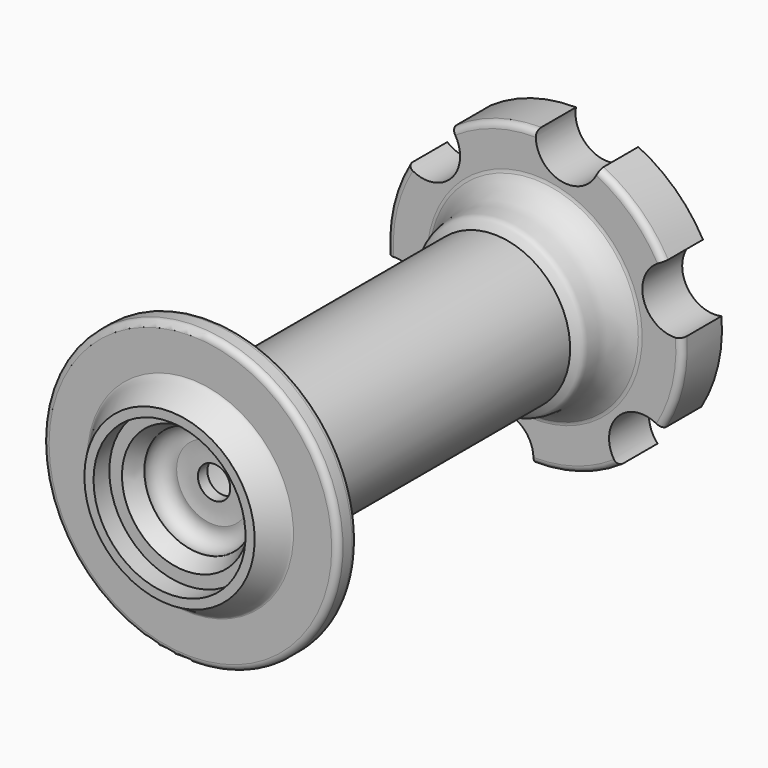
from build123d import *

# Parameters (mm, degrees)
F2_R          = 1
F4_R          = 5.0872245557
F5_DEPTH      = 25
F5_DEPTH_BACK = 25


# Not quite as in the source:
# - a feature names something its author has since deleted; it is built from what else it names


with BuildPart() as f1:
    # F0 (on Top) → F1 (revolve)
    with BuildSketch(Plane.XY):
        with BuildLine():
            Line((-12.045, 24.19), (-12.045, 0))
            Line((-12.045, 0), (-12.045, -24.19))
            add(Edge.make_bspline(
                [(-12.045, -24.19), (-12.5958616321, -24.4968671697), (-13.7960381357, -25.0826911965), (-13.4774444038, -27.9229008757), (-15.2810031254, -31.3268076458), (-16.4584506699, -32.0230348179), (-16.8, -32.2)],
                knots=[0, 0, 0, 0, 0.2130240833, 0.4757651617, 0.7943682617, 1, 1, 1, 1], degree=3))
            Line((-16.8, -32.2), (-23.4, -32.2))
            Line((-23.4, -32.2), (-23.4, -36))
            Line((-23.4, -36), (-16.34, -36))
            add(Edge.make_bspline(
                [(-16.34, -36), (-16.0707529319, -35.9620323671), (-14.9726425226, -37.6439271493), (-14.3452255143, -38.6538248832), (-13.7752974798, -39.6449017449), (-13.5, -40.14)],
                knots=[0, 0, 0, 0, 0.3581062946, 0.6698519127, 1, 1, 1, 1], degree=3))
            Line((-13.5, -40.14), (-12.045, -40.14))
            Line((-12.045, -40.14), (-12.045, -37.01))
            Line((-12.045, -37.01), (-10.045, -37.01))
            add(Edge.make_bspline(
                [(-10.045, -37.01), (-9.4132699561, -35.9848800804), (-9.0350072413, -35.0615949654), (-8.684367441, -34.2704410489)],
                knots=[0, 0, 0, 0, 2.6156118111, 2.6156118111, 2.6156118111, 2.6156118111], degree=3))
            ThreePointArc((-8.684367441, -34.2704410489), (-8.0143701637, -32.0764184583), (-5.8012267005, -31.4725745291))
            add(Edge.make_bspline(
                [(-5.8012267005, -31.4725745291), (-5.0125441811, -31.2893478801), (-3.9752367105, -31.2296903089), (-2.5670640498, -31.31)],
                knots=[7.2710216109, 7.2710216109, 7.2710216109, 7.2710216109, 9.4026339966, 9.4026339966, 9.4026339966, 9.4026339966], degree=3))
            Line((-2.5670640498, -31.31), (-2.5670640498, -29.4319074601))
            Line((-2.5670640498, -29.4319074601), (-9.8987429366, -29.4319074601))
            Line((-9.8987429366, -29.4319074601), (-9.8987429366, 0))
            Line((-9.8987429366, 0), (-9.8987429366, 29.4319074601))
            Line((-9.8987429366, 29.4319074601), (-4, 29.4319074601))
            Line((-4, 29.4319074601), (-4, 31.8579636514))
            Line((-4, 31.8579636514), (-8.9853084335, 31.8579636514))
            ThreePointArc((-8.9853084335, 31.8579636514), (-9.7346235261, 32.1683401253), (-10.045, 32.9176552179))
            Line((-10.045, 32.9176552179), (-10.045, 37.01))
            Line((-10.045, 37.01), (-12.045, 37.01))
            Line((-12.045, 37.01), (-12.045, 40.14))
            Line((-12.045, 40.14), (-23.4, 40.0790013373))
            Line((-23.4, 40.0790013373), (-23.4, 32.2))
            Line((-23.4, 32.2), (-16.8, 32.2))
            add(Edge.make_bspline(
                [(-12.045, 24.19), (-12.5958616321, 24.4968671697), (-13.7960381357, 25.0826911965), (-13.4774444038, 27.9229008757), (-15.2810031254, 31.3268076458), (-16.4584506699, 32.0230348179), (-16.8, 32.2)],
                knots=[0, 0, 0, 0, 0.2130240833, 0.4757651617, 0.7943682617, 1, 1, 1, 1], degree=3))
        make_face()
    revolve(axis=Axis((0, 20.07, 0), (0, 1, 0)))

    # F2
    f2_edges = [f1.edges().sort_by_distance(p)[0] for p in [
        (23.4, -32.2, 0),
        (23.4, -36, 0),
        (23.4, 32.2, 0),
        (16.8, 32.2, 0),
    ]]
    fillet(f2_edges, radius=F2_R)

    # F4 (on plane+point) → F5 (cut, two sides)
    with BuildSketch(Plane.XZ.offset(-40.0790013373)) as f5_sk:
        with Locations((-5.2686650306, -22.5467141718)):
            Circle(F4_R)
        with Locations((16.8916947293, -15.8361548464)):
            Circle(F4_R)
        with Locations((22.1603597599, 6.7105593254)):
            Circle(F4_R)
        with Locations((5.2686650306, 22.5467141718)):
            Circle(F4_R)
        with Locations((-16.8916947293, 15.8361548464)):
            Circle(F4_R)
        with Locations((-22.1603597599, -6.7105593254)):
            Circle(F4_R)
    extrude(amount=F5_DEPTH, mode=Mode.SUBTRACT)
    extrude(f5_sk.sketch, amount=-F5_DEPTH_BACK, mode=Mode.SUBTRACT)


solid = f1.part
